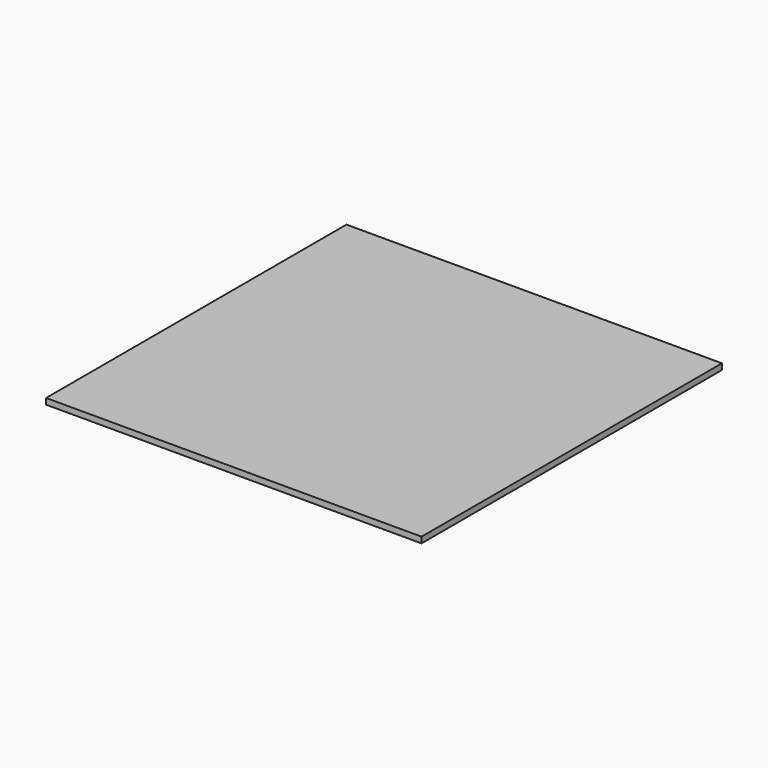
from build123d import *

# Parameters (mm, degrees)
F0_W     = 200
F0_H     = 200
F1_DEPTH = 3.175


# Not quite as in the source:
# - a length typed as a fraction of an inch, garbled in the dataset ("3 / 203.2 mm" for 3/8 in), is restored


with BuildPart() as f1:
    # F0 (on Top) → F1 (new body)
    with BuildSketch(Plane.XY):
        Rectangle(F0_W, F0_H)
    extrude(amount=F1_DEPTH)


solid = f1.part
